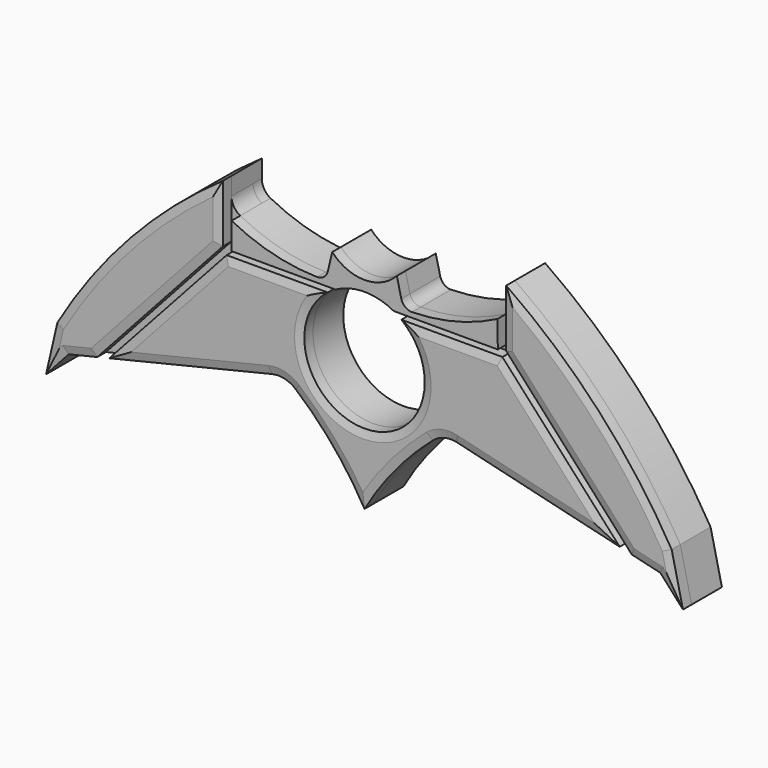
from build123d import *
from build123d import SkipClean  # not in build123d's __all__

# Parameters (mm, degrees)
F0_R                   = 11.1329203893
F1_DEPTH               = 2
F3_DEPTH               = 7
F5_DEPTH               = 0.4
DRAFT_F5_DRAFTED_ANGLE = 75
F7_DEPTH               = 0.4
DRAFT_F7_DRAFTED_ANGLE = 75
F9_DEPTH               = 0.4
DRAFT_F9_DRAFTED_ANGLE = 75
F10_DEPTH              = 7


# Not quite as in the source:
# - an extrude with a draft is written as a straight extrude whose walls are then drafted


with BuildPart() as f1:
    # F0 (on Front) → F1 (new body)
    with BuildSketch(Plane.XZ):
        with BuildLine():
            Line((54.6900890768, -4.4757057913), (58.8746277001, -9.1011243481))
            Line((58.8746277001, -9.1011243481), (56.7823583885, 0))
            ThreePointArc((56.7823583885, 0), (43.2885624533, 18.1760139058), (26.1943303049, 33.0164059997))
            Line((26.1943303049, 33.0164059997), (26.1943303049, 29.7207321387))
            Line((26.1943303049, 29.7207321387), (26.1943303049, 27.9525234479))
            ThreePointArc((26.1943303049, 27.9525234479), (25.3917782232, 27.4952000401), (24.5777001445, 27.0587238954))
            ThreePointArc((24.5777001445, 27.0587238954), (16.9116516132, 24.1340015075), (8.7811709074, 23.0305593378))
            ThreePointArc((8.7811709074, 23.0305593378), (7.9717977828, 23.0234333522), (7.1624702929, 23.0345979651))
            Line((7.1624702929, 23.0345979651), (6.7960089309, 24.5641755202))
            Line((6.7960089309, 24.5641755202), (5.9707658365, 28.0086677521))
            ThreePointArc((5.9707658365, 28.0086677521), (0, 25.4116508554), (-5.9707658365, 28.0086677521))
            Line((-5.9707658365, 28.0086677521), (-6.7960089309, 24.5641755202))
            ThreePointArc((-6.7960089309, 24.5641755202), (-7.518258282, 23.4474414872), (-8.7811709074, 23.0305593378))
            ThreePointArc((-8.7811709074, 23.0305593378), (-16.9116516132, 24.1340015075), (-24.5777001445, 27.0587238954))
            ThreePointArc((-24.5777001445, 27.0587238954), (-25.7585172636, 28.1635085707), (-26.1943303049, 29.7207321387))
            Line((-26.1943303049, 29.7207321387), (-26.1943303049, 33.0164059997))
            ThreePointArc((-26.1943303049, 33.0164059997), (-43.2885624533, 18.1760139058), (-56.7823583885, 0))
            Line((-56.7823583885, 0), (-58.8746277001, -9.1011243481))
            Line((-58.8746277001, -9.1011243481), (-54.6900890768, -4.4757057913))
            Line((-54.6900890768, -4.4757057913), (-17.1127793183, 4.5271931256))
            ThreePointArc((-17.1127793183, 4.5271931256), (-14.7862683626, 4.5280034697), (-12.7112426695, 3.4758997408))
            ThreePointArc((-12.7112426695, 3.4758997408), (-5.684214863, -3.6358963853), (0, -11.8606435135))
            ThreePointArc((0, -11.8606435135), (5.6979334186, -3.6539375678), (12.7098947356, 3.4628641164))
            ThreePointArc((12.7098947356, 3.4628641164), (14.7893408453, 4.5235207676), (17.1236689122, 4.5245841598))
            Line((17.1236689122, 4.5245841598), (54.6900890768, -4.4757057913))
        make_face()
        with Locations((0, 12.3495897278)):
            Circle(F0_R, mode=Mode.SUBTRACT)
        with BuildLine():
            Line((26.1943303049, 27.9525234479), (26.1943303049, 29.7207321387))
            ThreePointArc((26.1943303049, 29.7207321387), (25.7585172636, 28.1635085707), (24.5777001445, 27.0587238954))
            ThreePointArc((24.5777001445, 27.0587238954), (25.3917782232, 27.4952000401), (26.1943303049, 27.9525234479))
        make_face()
        with BuildLine():
            ThreePointArc((7.1624702929, 23.0345979651), (7.9717977828, 23.0234333522), (8.7811709074, 23.0305593378))
            ThreePointArc((8.7811709074, 23.0305593378), (7.518258282, 23.4474414872), (6.7960089309, 24.5641755202))
            Line((6.7960089309, 24.5641755202), (7.1624702929, 23.0345979651))
        make_face()
    extrude(amount=F1_DEPTH)

    # F2 (on face) → F3 (join)
    with BuildSketch(Plane.XZ.offset(2)):
        with BuildLine():
            ThreePointArc((11.1329203893, 12.3495897278), (-4.907473906, 2.3566614154), (-6.8064185738, 21.1595036089))
            Line((-6.8064185738, 21.1595036089), (-25.4939251943, 21.1595036089))
            Line((-25.4939251943, 21.1595036089), (-47.1803539642, -2.6764980634))
            Line((-47.1803539642, -2.6764980634), (-17.1127793183, 4.5271931256))
            ThreePointArc((-17.1127793183, 4.5271931256), (-14.7862683626, 4.5280034697), (-12.7112426695, 3.4758997408))
            ThreePointArc((-12.7112426695, 3.4758997408), (-5.684214863, -3.6358963853), (0, -11.8606435135))
            ThreePointArc((0, -11.8606435135), (5.6979334186, -3.6539375678), (12.7098947356, 3.4628641164))
            ThreePointArc((12.7098947356, 3.4628641164), (14.7893408453, 4.5235207676), (17.1236689122, 4.5245841598))
            Line((17.1236689122, 4.5245841598), (47.1803539642, -2.6764980634))
            Line((47.1803539642, -2.6764980634), (25.4939251943, 21.1595036089))
            Line((25.4939251943, 21.1595036089), (6.8064185738, 21.1595036089))
            ThreePointArc((6.8064185738, 21.1595036089), (9.9929283124, 17.2570636338), (11.1329203893, 12.3495897278))
        make_face()
        with BuildLine():
            ThreePointArc((-8.7811709074, 23.0305593378), (-16.9116516132, 24.1340015075), (-24.5777001445, 27.0587238954))
            Line((-24.5777001445, 27.0587238954), (-24.5777001445, 22.101605311))
            Line((-24.5777001445, 22.101605311), (-5.370298731, 22.101605311))
            ThreePointArc((-5.370298731, 22.101605311), (0, 23.4825101171), (5.370298731, 22.101605311))
            Line((5.370298731, 22.101605311), (24.6434782032, 22.101605311))
            Line((24.6434782032, 22.101605311), (24.5777001445, 27.0587238954))
            ThreePointArc((24.5777001445, 27.0587238954), (16.9116516132, 24.1340015075), (8.7811709074, 23.0305593378))
            ThreePointArc((8.7811709074, 23.0305593378), (7.518258282, 23.4474414872), (6.7960089309, 24.5641755202))
            Line((6.7960089309, 24.5641755202), (5.9707658365, 28.0086677521))
            ThreePointArc((5.9707658365, 28.0086677521), (0, 25.4116508554), (-5.9707658365, 28.0086677521))
            Line((-5.9707658365, 28.0086677521), (-6.7960089309, 24.5641755202))
            ThreePointArc((-6.7960089309, 24.5641755202), (-7.518258282, 23.4474414872), (-8.7811709074, 23.0305593378))
        make_face()
        with BuildLine():
            Line((-26.1943303049, 22.35221304), (-26.1943303049, 29.7207321387))
            Line((-26.1943303049, 29.7207321387), (-26.1943303049, 33.0164059997))
            ThreePointArc((-26.1943303049, 33.0164059997), (-43.2885624533, 18.1760139058), (-56.7823583885, 0))
            Line((-56.7823583885, 0), (-58.8746277001, -9.1011243481))
            Line((-58.8746277001, -9.1011243481), (-54.6900890768, -4.4757057913))
            Line((-54.6900890768, -4.4757057913), (-49.4011765897, -3.2085702564))
            Line((-49.4011765897, -3.2085702564), (-26.1943303049, 22.35221304))
        make_face()
        with BuildLine():
            Line((26.1943303049, 33.0164059997), (26.1943303049, 29.7207321387))
            Line((26.1943303049, 29.7207321387), (26.1943303049, 22.35221304))
            Line((26.1943303049, 22.35221304), (49.4011765897, -3.2085702564))
            Line((49.4011765897, -3.2085702564), (54.6900890768, -4.4757057913))
            Line((54.6900890768, -4.4757057913), (58.8746277001, -9.1011243481))
            Line((58.8746277001, -9.1011243481), (56.7823583885, 0))
            ThreePointArc((56.7823583885, 0), (43.2885624533, 18.1760139058), (26.1943303049, 33.0164059997))
        make_face()
    extrude(amount=F3_DEPTH)


with BuildPart() as f5_drafted:
    # F4 (on face) → F5 (new body)
    with BuildSketch(Plane.XZ.offset(9)):
        with BuildLine():
            Line((25.4939251943, 21.1595036089), (6.8064185738, 21.1595036089))
            ThreePointArc((6.8064185738, 21.1595036089), (0, 1.2166693385), (-6.8064185738, 21.1595036089))
            Line((-6.8064185738, 21.1595036089), (-25.4939251943, 21.1595036089))
            Line((-25.4939251943, 21.1595036089), (-47.1803539642, -2.6764980634))
            Line((-47.1803539642, -2.6764980634), (-17.1127793183, 4.5271931256))
            ThreePointArc((-17.1127793183, 4.5271931256), (-14.7862683626, 4.5280034697), (-12.7112426695, 3.4758997408))
            ThreePointArc((-12.7112426695, 3.4758997408), (-5.684214863, -3.6358963853), (0, -11.8606435135))
            ThreePointArc((0, -11.8606435135), (5.6979334186, -3.6539375678), (12.7098947356, 3.4628641164))
            ThreePointArc((12.7098947356, 3.4628641164), (14.7893408453, 4.5235207676), (17.1236689122, 4.5245841598))
            Line((17.1236689122, 4.5245841598), (47.1803539642, -2.6764980634))
            Line((47.1803539642, -2.6764980634), (25.4939251943, 21.1595036089))
        make_face()
    extrude(amount=F5_DEPTH)

    # draft_F5_drafted
    draft_f5_drafted_walls = [f5_drafted.faces().sort_by_distance(p)[0] for p in [
        (32.1520114382, -9.2666666667, 0.9240430482),
        (36.3371395792, -9.2666666667, 9.2415027728),
        (16.150171884, -9.2666666667, 21.1595036089),
        (0, -9.2666666667, 1.2166693385),
        (-16.150171884, -9.2666666667, 21.1595036089),
        (-36.3371395792, -9.2666666667, 9.2415027728),
        (-32.1465666412, -9.2666666667, 0.9253475311),
        (-14.7862683626, -9.2666666667, 4.5280034697),
        (-5.684214863, -9.2666666667, -3.6358963853),
        (5.6979334186, -9.2666666667, -3.6539375678),
        (14.7893408453, -9.2666666667, 4.5235207676),
    ]]
    draft(draft_f5_drafted_walls, neutral_plane=Plane.XZ.offset(9), angle=DRAFT_F5_DRAFTED_ANGLE)


with BuildPart() as f1_1:
    add(f1.part, clean=False)

    # join_F5_drafted: union F5_drafted
    add(f5_drafted.part)


with BuildPart() as f7_drafted:
    # F6 (on face) → F7 (new body)
    with BuildSketch(Plane.XZ.offset(9)):
        with BuildLine():
            Line((-56.7823583885, 0), (-58.8746277001, -9.1011243481))
            Line((-58.8746277001, -9.1011243481), (-54.6900890768, -4.4757057913))
            Line((-54.6900890768, -4.4757057913), (-49.4011765897, -3.2085702564))
            Line((-49.4011765897, -3.2085702564), (-26.1943303049, 22.35221304))
            Line((-26.1943303049, 22.35221304), (-26.1943303049, 33.0164059997))
            ThreePointArc((-26.1943303049, 33.0164059997), (-43.2885624533, 18.1760139058), (-56.7823583885, 0))
        make_face()
    extrude(amount=F7_DEPTH)

    # draft_F7_drafted
    draft_f7_drafted_walls = [f7_drafted.faces().sort_by_distance(p)[0] for p in [
        (-57.8284930443, -9.2666666667, -4.550562174),
        (-56.7823583885, -9.2666666667, -6.7884150697),
        (-52.0456328332, -9.2666666667, -3.8421380238),
        (-37.7977534473, -9.2666666667, 9.5718213918),
        (-26.1943303049, -9.2666666667, 27.6843095198),
        (-43.2885624533, -9.2666666667, 18.1760139058),
    ]]
    draft(draft_f7_drafted_walls, neutral_plane=Plane.XZ.offset(9), angle=DRAFT_F7_DRAFTED_ANGLE)


with BuildPart() as f1_2:
    add(f1_1.part, clean=False)

    # join_F7_drafted: union F7_drafted
    add(f7_drafted.part)


with BuildPart() as f9_drafted:
    # F8 (on face) → F9 (new body)
    with BuildSketch(Plane.XZ.offset(9)):
        with BuildLine():
            Line((54.6900890768, -4.4757057913), (58.8746277001, -9.1011243481))
            Line((58.8746277001, -9.1011243481), (56.7823583885, 0))
            ThreePointArc((56.7823583885, 0), (43.2885624533, 18.1760139058), (26.1943303049, 33.0164059997))
            Line((26.1943303049, 33.0164059997), (26.1943303049, 22.35221304))
            Line((26.1943303049, 22.35221304), (49.4011765897, -3.2085702564))
            Line((49.4011765897, -3.2085702564), (54.6900890768, -4.4757057913))
        make_face()
    extrude(amount=F9_DEPTH)

    # draft_F9_drafted
    draft_f9_drafted_walls = [f9_drafted.faces().sort_by_distance(p)[0] for p in [
        (56.7823583885, -9.2666666667, -6.7884150697),
        (57.8284930443, -9.2666666667, -4.550562174),
        (43.2885624533, -9.2666666667, 18.1760139058),
        (26.1943303049, -9.2666666667, 27.6843095198),
        (37.7977534473, -9.2666666667, 9.5718213918),
        (52.0456328332, -9.2666666667, -3.8421380238),
    ]]
    draft(draft_f9_drafted_walls, neutral_plane=Plane.XZ.offset(9), angle=DRAFT_F9_DRAFTED_ANGLE)


with BuildPart() as f1_3:
    add(f1_2.part, clean=False)

    # join_F9_drafted: union F9_drafted
    add(f9_drafted.part)

    # F0 (on Front) → F10 (join)
    with BuildSketch(Plane.XZ):
        with BuildLine():
            Line((54.6900890768, -4.4757057913), (58.8746277001, -9.1011243481))
            Line((58.8746277001, -9.1011243481), (56.7823583885, 0))
            ThreePointArc((56.7823583885, 0), (43.2885624533, 18.1760139058), (26.1943303049, 33.0164059997))
            Line((26.1943303049, 33.0164059997), (26.1943303049, 29.7207321387))
            Line((26.1943303049, 29.7207321387), (26.1943303049, 27.9525234479))
            ThreePointArc((26.1943303049, 27.9525234479), (25.3917782232, 27.4952000401), (24.5777001445, 27.0587238954))
            ThreePointArc((24.5777001445, 27.0587238954), (16.9116516132, 24.1340015075), (8.7811709074, 23.0305593378))
            ThreePointArc((8.7811709074, 23.0305593378), (7.9717977828, 23.0234333522), (7.1624702929, 23.0345979651))
            Line((7.1624702929, 23.0345979651), (6.7960089309, 24.5641755202))
            Line((6.7960089309, 24.5641755202), (5.9707658365, 28.0086677521))
            ThreePointArc((5.9707658365, 28.0086677521), (0, 25.4116508554), (-5.9707658365, 28.0086677521))
            Line((-5.9707658365, 28.0086677521), (-6.7960089309, 24.5641755202))
            ThreePointArc((-6.7960089309, 24.5641755202), (-7.518258282, 23.4474414872), (-8.7811709074, 23.0305593378))
            ThreePointArc((-8.7811709074, 23.0305593378), (-16.9116516132, 24.1340015075), (-24.5777001445, 27.0587238954))
            ThreePointArc((-24.5777001445, 27.0587238954), (-25.7585172636, 28.1635085707), (-26.1943303049, 29.7207321387))
            Line((-26.1943303049, 29.7207321387), (-26.1943303049, 33.0164059997))
            ThreePointArc((-26.1943303049, 33.0164059997), (-43.2885624533, 18.1760139058), (-56.7823583885, 0))
            Line((-56.7823583885, 0), (-58.8746277001, -9.1011243481))
            Line((-58.8746277001, -9.1011243481), (-54.6900890768, -4.4757057913))
            Line((-54.6900890768, -4.4757057913), (-17.1127793183, 4.5271931256))
            ThreePointArc((-17.1127793183, 4.5271931256), (-14.7862683626, 4.5280034697), (-12.7112426695, 3.4758997408))
            ThreePointArc((-12.7112426695, 3.4758997408), (-5.684214863, -3.6358963853), (0, -11.8606435135))
            ThreePointArc((0, -11.8606435135), (5.6979334186, -3.6539375678), (12.7098947356, 3.4628641164))
            ThreePointArc((12.7098947356, 3.4628641164), (14.7893408453, 4.5235207676), (17.1236689122, 4.5245841598))
            Line((17.1236689122, 4.5245841598), (54.6900890768, -4.4757057913))
        make_face()
        with Locations((0, 12.3495897278)):
            Circle(F0_R, mode=Mode.SUBTRACT)
        with BuildLine():
            Line((26.1943303049, 27.9525234479), (26.1943303049, 29.7207321387))
            ThreePointArc((26.1943303049, 29.7207321387), (25.7585172636, 28.1635085707), (24.5777001445, 27.0587238954))
            ThreePointArc((24.5777001445, 27.0587238954), (25.3917782232, 27.4952000401), (26.1943303049, 27.9525234479))
        make_face()
        with BuildLine():
            ThreePointArc((7.1624702929, 23.0345979651), (7.9717977828, 23.0234333522), (8.7811709074, 23.0305593378))
            ThreePointArc((8.7811709074, 23.0305593378), (7.518258282, 23.4474414872), (6.7960089309, 24.5641755202))
            Line((6.7960089309, 24.5641755202), (7.1624702929, 23.0345979651))
        make_face()
    with SkipClean():  # cleaning this boolean's faces spoils the solid; the shape is the same uncleaned
        extrude(amount=F10_DEPTH)


solid = f1_3.part
